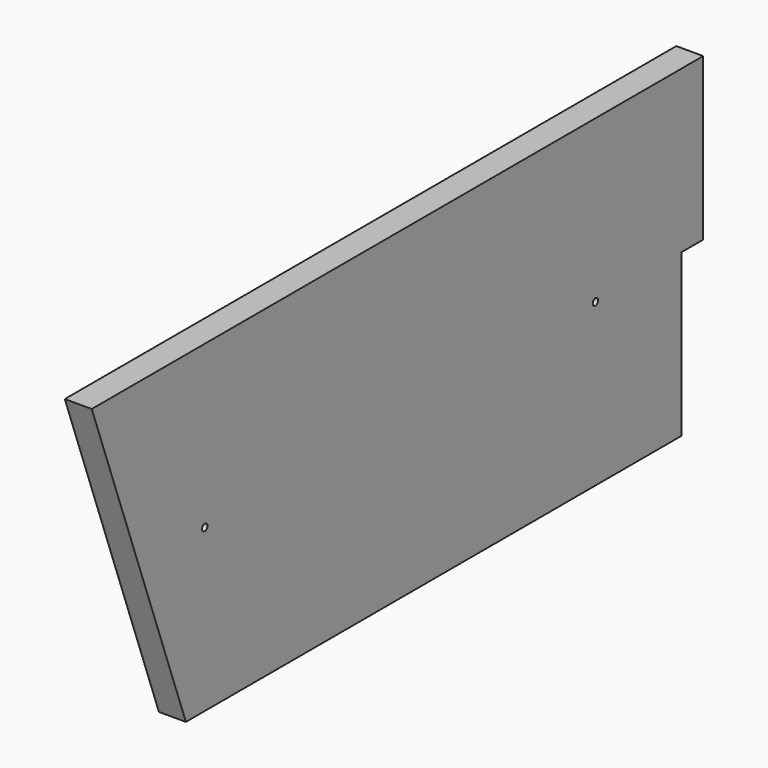
from build123d import *

# Parameters (mm, degrees)
F2_DEPTH = 12.7
F3_R     = 1.5875
F4_DEPTH = 12.701


# Not quite as in the source:
# - a feature names something its author has since deleted; it is built from what else it names


with BuildPart() as f2:
    # F1 (on face) → F2 (new body)
    with BuildSketch(Plane.YZ):
        Polygon((-152.4, -76.2), (139.7, -76.2), (139.7, 0), (152.4, 0), (152.4, 76.2), (-152.4, 76.2), (-207.8690637022, 76.2), align=None)
    extrude(amount=F2_DEPTH)

    # F3 (on face) → F4 (cut, through all)
    with BuildSketch(Plane.YZ):
        with Locations((-141.2875, 0)):
            Circle(F3_R)
        with Locations((88.9, 0)):
            Circle(F3_R)
    extrude(amount=F4_DEPTH, mode=Mode.SUBTRACT)


solid = f2.part
